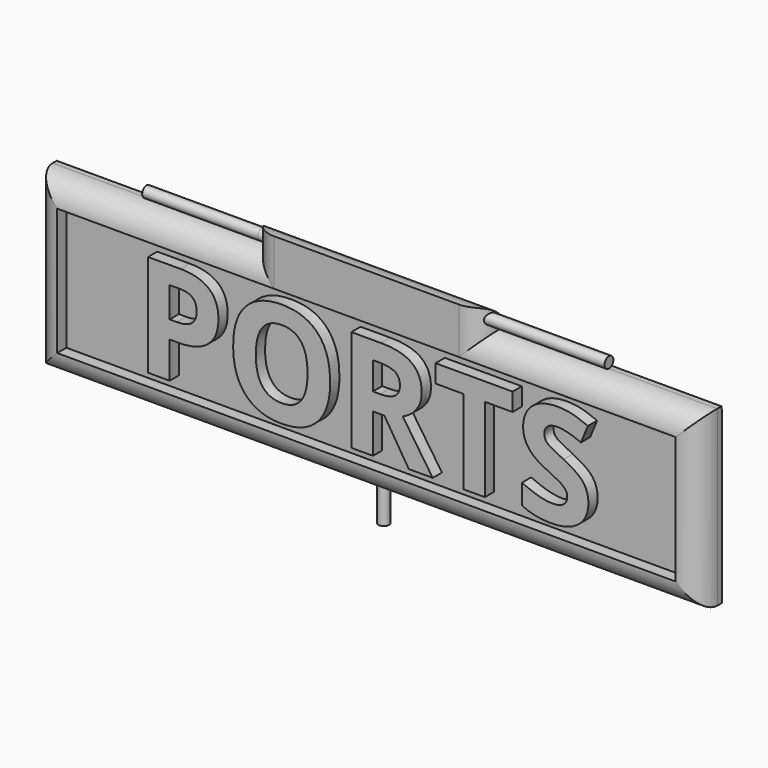
from build123d import *

# Parameters (mm, degrees)
F0_W          = 73.025
F0_H          = 19.05
F1_DEPTH      = 3.175
F2_R          = 0.5969
F3_DEPTH      = 3.81
F4_W          = 25.4
F4_H          = 3.175
F5_DEPTH      = 2.54
F6_R          = 3.17499
F7_R          = 0.6025929155
F8_DEPTH      = 12.7
F9_R          = 0.5983755032
F10_DEPTH     = 12.7
F11_T1_DEPTH  = 31.75
F11_T3_DEPTH  = 30.1625
F11_T5_DEPTH  = 30.1625
F11_T10_DEPTH = 85.725
F11_S11_R     = 0.5969
F11_T12_DEPTH = 44
F11_T16_DEPTH = 8.89
F11_S17_R     = 0.6025929155
F11_T18_DEPTH = 6
F11_T22_DEPTH = 8.89
F11_S23_R     = 0.5983755032
F11_T24_DEPTH = 6
F11_T29_DEPTH = 36.5125
F11_T33_DEPTH = 15.24
F11_T40_DEPTH = 15.24
F11_T44_DEPTH = 36.5125
F12_W         = 67.945
F12_H         = 13.97
F13_DEPTH     = 1.27
F14_TEXT_SIZE = 15.6827938836
F15_DEPTH     = 1.27


# Not quite as in the source:
# - a fillet or chamfer that OpenCascade refuses, or shapes differently, is made with other operations: its cross-section is extruded or revolved along the edge and cut away or added
# - a fillet or chamfer is up to 0.001 mm smaller than in the source, because OpenCascade refuses the exact size
# - Text() gives the source's letters only with a copy of the font that has no kerning and outlines rounded to 1/6400 em; it was checked with that copy


with BuildPart() as f1:
    # F0 (on Front) → F1 (new body)
    with BuildSketch(Plane.XZ):
        with Locations((-21.1988968721, 8.4669439821)):
            Rectangle(F0_W, F0_H)
    extrude(amount=F1_DEPTH)

    # F2 (on face) → F3 (join)
    with BuildSketch(Plane(origin=(0, 0, -1.0580560179), x_dir=(1, 0, 0), z_dir=(0, 0, -1))):
        with Locations((-21.1988968721, 0.79375)):
            Circle(F2_R)
    extrude(amount=F3_DEPTH)

    # F4 (on face) → F5 (join)
    with BuildSketch(Plane.XY.offset(17.9919439821)):
        with Locations((-21.1988968721, -1.5875)):
            Rectangle(F4_W, F4_H)
    extrude(amount=F5_DEPTH)

    # F6 (radius 3.175 in the source; OpenCascade refuses exactly that, so slightly less here)
    f6_edges = [f1.edges().sort_by_distance(p)[0] for p in [
        (-21.198897, 0, 20.531944),
    ]]
    fillet(f6_edges, radius=F6_R)

    # F7 (on face) → F8 (join)
    with BuildSketch(Plane.YZ.offset(-8.4988968721)):
        with Locations((-1.6195740133, 19.2619439821)):
            Circle(F7_R)
    extrude(amount=F8_DEPTH)

    # F9 (on face) → F10 (join)
    with BuildSketch(Plane(origin=(-33.8988968721, 0, 0), x_dir=(0, -1, 0), z_dir=(-1, 0, 0))):
        with Locations((1.6195740133, 19.2619439821)):
            Circle(F9_R)
    extrude(amount=F10_DEPTH)

    # F11: fillet of radius 2.54 on 7 edges, made by hand

    # F11_s2 → F11_t1 (cut)
    with BuildSketch(Plane.XY.offset(-7.4080560179)):
        with BuildLine():
            ThreePointArc((12.7736031279, -3.175), (14.5696543522, -2.4310512242), (15.3136031279, -0.635))
            Line((15.3136031279, -0.635), (15.3136031279, -3.175))
            Line((15.3136031279, -3.175), (12.7736031279, -3.175))
        make_face()
        with BuildLine():
            ThreePointArc((-55.1713968721, -3.175), (-56.9674480963, -2.4310512242), (-57.7113968721, -0.635))
            Line((-57.7113968721, -0.635), (-57.7113968721, -3.175))
            Line((-57.7113968721, -3.175), (-55.1713968721, -3.175))
        make_face()
    extrude(amount=F11_T1_DEPTH, mode=Mode.SUBTRACT)

    # F11_s4 → F11_t3 (cut)
    with BuildSketch(Plane.YZ.offset(-8.4988968721)):
        with BuildLine():
            ThreePointArc((-0.635, 17.9919439821), (-2.4310512242, 17.2479952063), (-3.175, 15.4519439821))
            Line((-3.175, 15.4519439821), (-3.175, 17.9919439821))
            Line((-3.175, 17.9919439821), (-0.635, 17.9919439821))
        make_face()
    extrude(amount=F11_T3_DEPTH, mode=Mode.SUBTRACT)

    # F11_s6 → F11_t5 (cut)
    with BuildSketch(Plane.YZ.offset(-64.0613968721)):
        with BuildLine():
            ThreePointArc((-3.175, 15.4519439821), (-2.4310512242, 17.2479952063), (-0.635, 17.9919439821))
            Line((-0.635, 17.9919439821), (-3.175, 17.9919439821))
            Line((-3.175, 17.9919439821), (-3.175, 15.4519439821))
        make_face()
    extrude(amount=F11_T5_DEPTH, mode=Mode.SUBTRACT)


with BuildPart() as f11_tool8:
    # F11_s9 → F11_t10 (new body)
    with BuildSketch(Plane.YZ.offset(-64.0613968721)):
        with BuildLine():
            ThreePointArc((-3.175, 1.4819439821), (-2.4310512242, -0.3141072422), (-0.635, -1.0580560179))
            Line((-0.635, -1.0580560179), (-3.175, -1.0580560179))
            Line((-3.175, -1.0580560179), (-3.175, 1.4819439821))
        make_face()
    extrude(amount=F11_T10_DEPTH)

    # F11_s11 → F11_t12 (cut, symmetric)
    with BuildSketch(Plane.XY.offset(0.2)):
        with Locations((-21.1988968721, -0.79375)):
            Circle(F11_S11_R)
    extrude(amount=F11_T12_DEPTH, both=True, mode=Mode.SUBTRACT)


with BuildPart() as f1_1:
    add(f1.part)

    # F11_t7: cut F11_tool8
    add(f11_tool8.part, mode=Mode.SUBTRACT)


with BuildPart() as f11_tool14:
    # F11_s15 → F11_t16 (new body)
    with BuildSketch(Plane.XY.offset(17.9919439821)):
        with BuildLine():
            ThreePointArc((-8.4988968721, -0.635), (-9.2428456478, -2.4310512242), (-11.0388968721, -3.175))
            Line((-11.0388968721, -3.175), (-8.4988968721, -3.175))
            Line((-8.4988968721, -3.175), (-8.4988968721, -0.635))
        make_face()
    extrude(amount=F11_T16_DEPTH)

    # F11_s17 → F11_t18 (cut, symmetric)
    with BuildSketch(Plane.YZ.offset(-9.8)):
        with Locations((-1.6195740133, 19.2619439821)):
            Circle(F11_S17_R)
    extrude(amount=F11_T18_DEPTH, both=True, mode=Mode.SUBTRACT)


with BuildPart() as f1_2:
    add(f1_1.part)

    # F11_t13: cut F11_tool14
    add(f11_tool14.part, mode=Mode.SUBTRACT)


with BuildPart() as f11_tool20:
    # F11_s21 → F11_t22 (new body)
    with BuildSketch(Plane.XY.offset(17.9919439821)):
        with BuildLine():
            ThreePointArc((-31.3588968721, -3.175), (-33.1549480963, -2.4310512242), (-33.8988968721, -0.635))
            Line((-33.8988968721, -0.635), (-33.8988968721, -3.175))
            Line((-33.8988968721, -3.175), (-31.3588968721, -3.175))
        make_face()
    extrude(amount=F11_T22_DEPTH)

    # F11_s23 → F11_t24 (cut, symmetric)
    with BuildSketch(Plane.YZ.offset(-32.6)):
        with Locations((-1.6195740133, 19.2619439821)):
            Circle(F11_S23_R)
    extrude(amount=F11_T24_DEPTH, both=True, mode=Mode.SUBTRACT)


with BuildPart() as f1_3:
    add(f1_2.part)

    # F11_t19: cut F11_tool20
    add(f11_tool20.part, mode=Mode.SUBTRACT)


with BuildPart() as f11_tool27:
    # F11_s28 → F11_t29 (new body)
    with BuildSketch(Plane.YZ.offset(21.6636031279)):
        with BuildLine():
            ThreePointArc((-0.635, 17.9919439821), (-2.4310512242, 17.2479952063), (-3.175, 15.4519439821))
            Line((-3.175, 15.4519439821), (-3.175, 17.9919439821))
            Line((-3.175, 17.9919439821), (-0.635, 17.9919439821))
        make_face()
    extrude(amount=-F11_T29_DEPTH)

    split(bisect_by=Plane.YZ.offset(-8.4988968721), keep=Keep.BOTTOM)


with BuildPart() as f11_tool31:
    # F11_s32 → F11_t33 (new body)
    with BuildSketch(Plane.XY.offset(11.6419439821)):
        with BuildLine():
            ThreePointArc((-8.4988968721, -0.635), (-9.2428456478, -2.4310512242), (-11.0388968721, -3.175))
            Line((-11.0388968721, -3.175), (-8.4988968721, -3.175))
            Line((-8.4988968721, -3.175), (-8.4988968721, -0.635))
        make_face()
    extrude(amount=F11_T33_DEPTH)

    split(bisect_by=Plane.XY.offset(17.9919439821), keep=Keep.BOTTOM)


with BuildPart() as f11_tool27_1:
    add(f11_tool27.part)

    # F11_t35: intersect F11_tool31
    add(f11_tool31.part, mode=Mode.INTERSECT)


with BuildPart() as f1_4:
    add(f1_3.part)

    # F11_t25: cut F11_tool27
    add(f11_tool27_1.part, mode=Mode.SUBTRACT)


with BuildPart() as f11_tool38:
    # F11_s39 → F11_t40 (new body)
    with BuildSketch(Plane.XY.offset(11.6419439821)):
        with BuildLine():
            ThreePointArc((-31.3588968721, -3.175), (-33.1549480963, -2.4310512242), (-33.8988968721, -0.635))
            Line((-33.8988968721, -0.635), (-33.8988968721, -3.175))
            Line((-33.8988968721, -3.175), (-31.3588968721, -3.175))
        make_face()
    extrude(amount=F11_T40_DEPTH)

    split(bisect_by=Plane.XY.offset(17.9919439821), keep=Keep.BOTTOM)


with BuildPart() as f11_tool42:
    # F11_s43 → F11_t44 (new body)
    with BuildSketch(Plane.YZ.offset(-27.5488968721)):
        with BuildLine():
            ThreePointArc((-3.175, 15.4519439821), (-2.4310512242, 17.2479952063), (-0.635, 17.9919439821))
            Line((-0.635, 17.9919439821), (-3.175, 17.9919439821))
            Line((-3.175, 17.9919439821), (-3.175, 15.4519439821))
        make_face()
    extrude(amount=-F11_T44_DEPTH)

    split(bisect_by=Plane.YZ.offset(-33.8988968721), keep=Keep.TOP)


with BuildPart() as f11_tool38_1:
    add(f11_tool38.part)

    # F11_t46: intersect F11_tool42
    add(f11_tool42.part, mode=Mode.INTERSECT)


with BuildPart() as f1_5:
    add(f1_4.part)

    # F11_t36: cut F11_tool38
    add(f11_tool38_1.part, mode=Mode.SUBTRACT)

    # F12 (on face) → F13 (cut)
    with BuildSketch(Plane.XZ.offset(3.175)):
        with Locations((-21.1988968721, 8.4669439821)):
            Rectangle(F12_W, F12_H)
    extrude(amount=-F13_DEPTH, mode=Mode.SUBTRACT)

    # F14 (on face) → F15 (join)
    with BuildSketch(Plane.XZ.offset(1.905)):
        with Locations((-46.5988968721, 2.8268323859)):
            Text('PORTS', F14_TEXT_SIZE, font='Open Sans', font_style=FontStyle.BOLD, text_align=(TextAlign.LEFT, TextAlign.BOTTOM))
    extrude(amount=F15_DEPTH)


solid = f1_5.part
